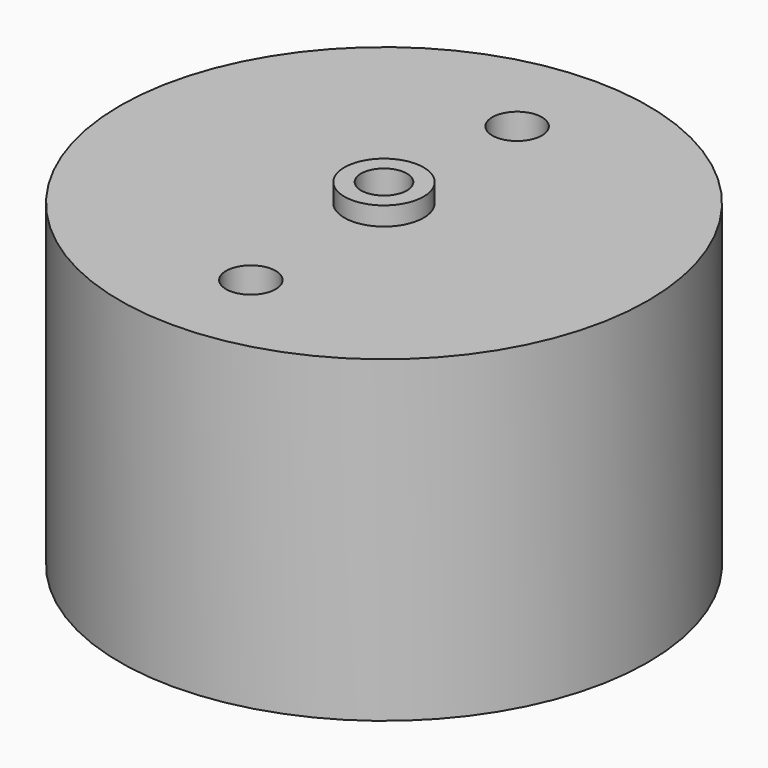
from build123d import *

# Parameters (mm, degrees)
F0_R     = 14.3848333842
F1_DEPTH = 17.3482
F4_R     = 2.159
F5_DEPTH = 1.016
F6_D     = 2.7051
F6_DEPTH = 5.87375
F6_TIP   = 0.8126940303
F8_D     = 2.5


# Not quite as in the source:
# - a feature names something its author has since deleted; it is built from what else it names


with BuildPart() as f1:
    # F0 (on Top) → F1 (new body)
    with BuildSketch(Plane.XY):
        Circle(F0_R)
    extrude(amount=F1_DEPTH)

    # F4 (on face) → F5 (join)
    with BuildSketch(Plane.XY.offset(17.3482)):
        Circle(F4_R)
    extrude(amount=F5_DEPTH)

    # F6
    with Locations(Plane.XY.offset(17.3482)):
        with Locations((0, 9.0678), (0, -9.0678)):
            Hole(F6_D / 2, depth=F6_DEPTH)
            with Locations((0, 0, -(F6_DEPTH + F6_TIP / 2))):  # 118° drill point
                Cone(0, F6_D / 2, F6_TIP, mode=Mode.SUBTRACT)

    # F8 (through all)
    with Locations(Plane.XY.offset(18.3642)):
        with Locations((0, 0)):
            Hole(F8_D / 2)


solid = f1.part
